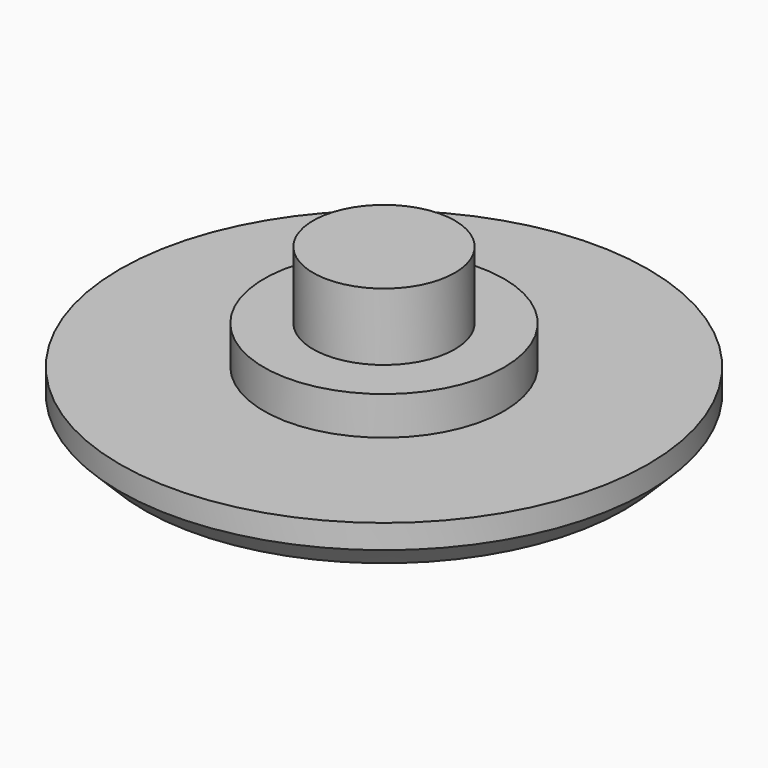
from build123d import *

# Parameters (mm, degrees)
F0_R     = 11
F0_R_2   = 5
F1_DEPTH = 2
F0_R_3   = 2.95
F2_DEPTH = 3.6
F0_R_4   = 1.8
F3_DEPTH = 6.4
F4_DEPTH = 1
F5_SIZE  = 1


# Not quite as in the source:
# - a fillet or chamfer that OpenCascade refuses, or shapes differently, is made with other operations: its cross-section is extruded or revolved along the edge and cut away or added
# - a feature of the source that left no trace in its solid (it failed there, or was rolled back) is left out


with BuildPart() as f1:
    # F0 (on Top) → F1 (new body)
    with BuildSketch(Plane.XY):
        Circle(F0_R)
        Circle(F0_R_2, mode=Mode.SUBTRACT)
    extrude(amount=F1_DEPTH)

    # F0 (on Top) → F2 (join)
    with BuildSketch(Plane.XY):
        Circle(F0_R_2)
        Circle(F0_R_3, mode=Mode.SUBTRACT)
    extrude(amount=F2_DEPTH)

    # F0 (on Top) → F3 (join)
    with BuildSketch(Plane.XY):
        Circle(F0_R_3)
        Circle(F0_R_4, mode=Mode.SUBTRACT)
        Circle(F0_R_4)
    extrude(amount=F3_DEPTH)

    # F0 (on Top) → F4 (cut)
    with BuildSketch(Plane.XY):
        Circle(F0_R_2)
        Circle(F0_R_3, mode=Mode.SUBTRACT)
        Circle(F0_R_3)
        Circle(F0_R_4, mode=Mode.SUBTRACT)
        Circle(F0_R_4)
    extrude(amount=F4_DEPTH, mode=Mode.SUBTRACT)

    # F5
    f5_edges = [f1.edges().sort_by_distance(p)[0] for p in [
        (-11, 0, 0),
    ]]
    chamfer(f5_edges, length=F5_SIZE)

    # F6: fillet of radius 10 on 1 edges, made by hand

    # F6_s1 → F6_t2 (revolve)
    with BuildSketch(Plane.XZ):
        with BuildLine():
            ThreePointArc((5, 0), (2.877169034, 0.7467943448), (0.6411010565, 1))
            Line((0.6411010565, 1), (5, 1))
            Line((5, 1), (5, 0))
        make_face()
    revolve(axis=Axis((0, 0, 1), (0, 0, 1)))


solid = f1.part
